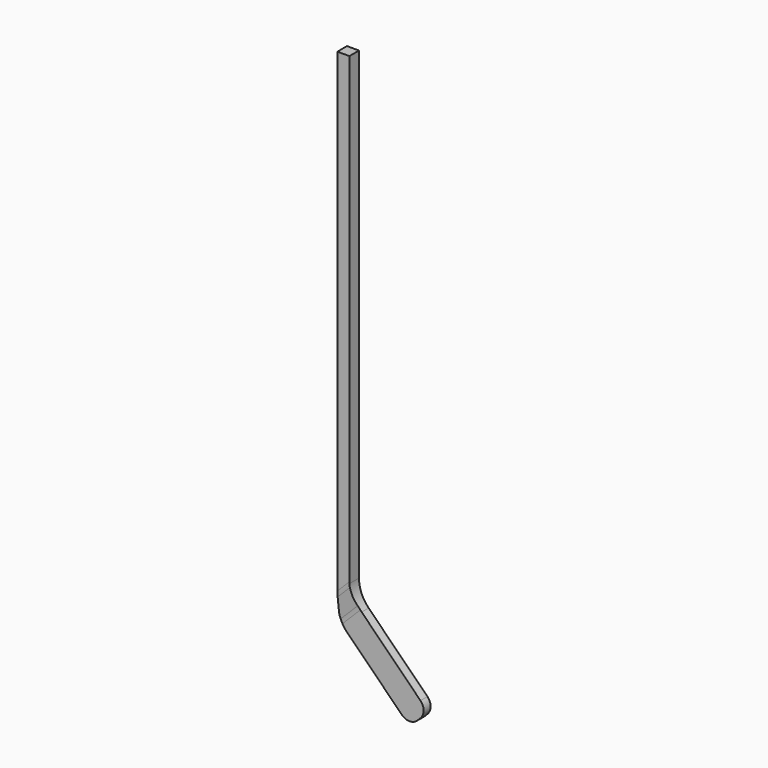
from build123d import *

# Parameters (mm, degrees)
F1_DEPTH    = 2.75
F2_T1_DEPTH = 30.499500005
F3_R        = 10
F6_DEPTH    = 31.7539349198
F7_R        = 15
F8_R        = 10


# Not quite as in the source:
# - a fillet or chamfer that OpenCascade refuses, or shapes differently, is made with other operations: its cross-section is extruded or revolved along the edge and cut away or added


with BuildPart() as f1:
    # F0 (on Front) → F1 (new body, symmetric)
    with BuildSketch(Plane.XZ):
        Polygon((0, 230), (0, 0), (31.8198051534, -31.8198051534), (40.3050865276, -23.3345237792), (5.5, 11.4705627485), (5.5, 230), align=None)
    extrude(amount=F1_DEPTH, both=True)

    # F2: fillet of radius 5 on 2 edges, made by hand

    # F2_s2 → F2_t1 (cut)
    with BuildSketch(Plane.XZ.offset(-15.2497500025)):
        with BuildLine():
            ThreePointArc((35.3553390593, -28.2844126688), (31.8198051534, -29.7488787629), (28.2842712475, -28.2844126688))
            Line((28.2842712475, -28.2844126688), (28.2135605693, -28.3551233469))
            ThreePointArc((28.2135605693, -28.3551233469), (29.9813628776, -30.1227842339), (31.7490944753, -31.8905158315))
            Line((31.7490944753, -31.8905158315), (31.8905158315, -31.8905158315))
            ThreePointArc((31.8905158315, -31.8905158315), (33.6582474291, -30.1227842339), (35.4260497374, -28.3551233469))
            Line((35.4260497374, -28.3551233469), (35.3553390593, -28.2844126688))
        make_face()
        with BuildLine():
            ThreePointArc((36.7696940431, -19.7989898732), (38.2341601371, -23.3345237792), (36.7696940431, -26.8700576851))
            Line((36.7696940431, -26.8700576851), (36.8404047212, -26.9407683632))
            ThreePointArc((36.8404047212, -26.9407683632), (38.6080656081, -25.1729660549), (40.3757972058, -23.4052344573))
            Line((40.3757972058, -23.4052344573), (40.3757972058, -23.263813101))
            ThreePointArc((40.3757972058, -23.263813101), (38.6080656081, -21.4960815034), (36.8404047212, -19.7282791951))
            Line((36.8404047212, -19.7282791951), (36.7696940431, -19.7989898732))
        make_face()
    extrude(amount=F2_T1_DEPTH, mode=Mode.SUBTRACT)

    # F3
    f3_edges = [f1.edges().sort_by_distance(p)[0] for p in [
        (0, 0, 0),
    ]]
    fillet(f3_edges, radius=F3_R)

    # F5 (on offset) → F6 (cut)
    with BuildSketch(Plane(origin=(0, 0, 0), x_dir=(0.7071067812, 0, -0.7071067812), z_dir=(-0.7071067812, 0, -0.7071067812))):
        Polygon((40, 2.75), (-8.2739908248, 2.75), (0.2329319046, 1.25), (45, 1.25), (45, 2.75), align=None)
    extrude(amount=-F6_DEPTH, mode=Mode.SUBTRACT)

    # F7
    f7_edges = [f1.edges().sort_by_distance(p)[0] for p in [
        (5.5, 0.357253, 11.470563),
    ]]
    fillet(f7_edges, radius=F7_R)

    # F8
    f8_edges = [f1.edges().sort_by_distance(p)[0] for p in [
        (2.753762, -2.75, 14.454952),
        (4.725257, -1.25, 4.395842),
    ]]
    fillet(f8_edges, radius=F8_R)


solid = f1.part
